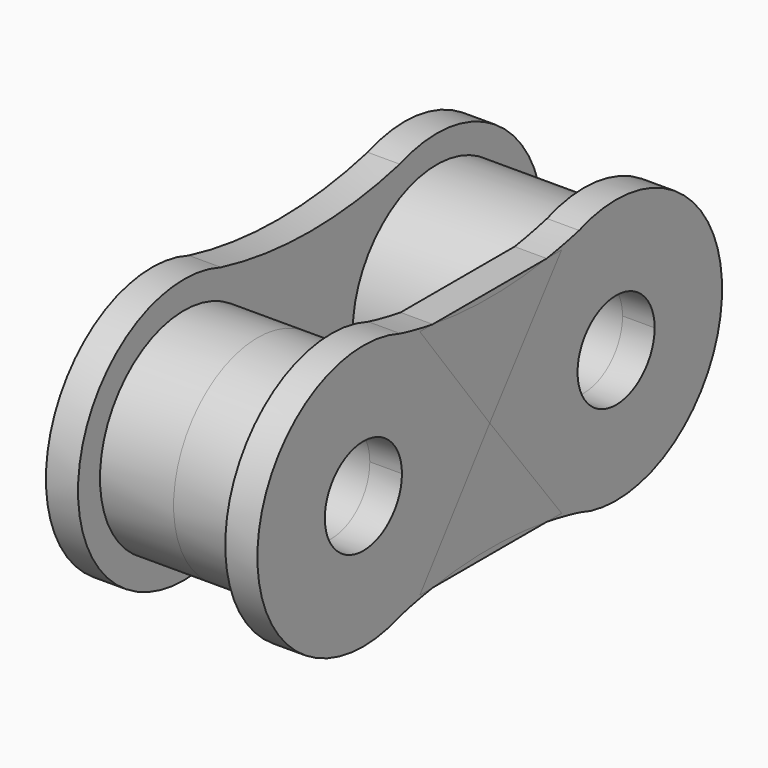
from build123d import *

# Parameters (mm, degrees)
F0_R     = 0.9144
F1_DEPTH = 0.3048
F2_R     = 1.9939
F2_R_2   = 0.9144
F3_DEPTH = 1.397
F8_DEPTH = 0.6096


# Not quite as in the source:
# - a pattern or mirror of a feature is missing from the dataset's text; its kind, count and spacing are read off the source's solid


with BuildPart() as f1:
    # F0 (on Right) → F1 (new body, symmetric)
    with BuildSketch(Plane.YZ):
        with BuildLine():
            ThreePointArc((2.1201945262, 2.3567084162), (0, 2.094238318), (-2.1201945262, 2.3567084162))
            ThreePointArc((-2.1201945262, 2.3567084162), (-5.5118, 0), (-2.1201945262, -2.3567084162))
            ThreePointArc((-2.1201945262, -2.3567084162), (0, -2.094238318), (2.1201945262, -2.3567084162))
            ThreePointArc((2.1201945262, -2.3567084162), (5.5118, 0), (2.1201945262, 2.3567084162))
        make_face()
        with Locations((-2.9972, 0)):
            Circle(F0_R, mode=Mode.SUBTRACT)
        with Locations((2.9972, 0)):
            Circle(F0_R, mode=Mode.SUBTRACT)
    extrude(amount=F1_DEPTH, both=True)

    # F2 (on face) → F3 (join)
    with BuildSketch(Plane.YZ.offset(0.3048)):
        with Locations((-2.9972, 0)):
            Circle(F2_R)
        with Locations((-2.9972, 0)):
            Circle(F2_R_2, mode=Mode.SUBTRACT)
    extrude(amount=F3_DEPTH)

    # F4: F1 across plane


with BuildPart() as f1_1:
    add(f1.part)
    add(f1.part.mirror(Plane.XZ))

    # F5: F1 across face


with BuildPart() as f1_2:
    add(f1_1.part)
    add(f1_1.part.mirror(Plane(origin=(1.7018, -2.9972, 0), x_dir=(0, 1, 0), z_dir=(1, 0, 0))))

    # F7 (on face) → F8 (join, through all)
    with BuildSketch(Plane.YZ.offset(3.7084)):
        Polygon((1.7045348049, -2.2), (0, 0), (-1.6570564457, -2.2), align=None)
    f8 = extrude(amount=-F8_DEPTH)

    # F8_copies: F8 across plane
    add(f8.mirror(Plane.XY))


solid = f1_2.part
